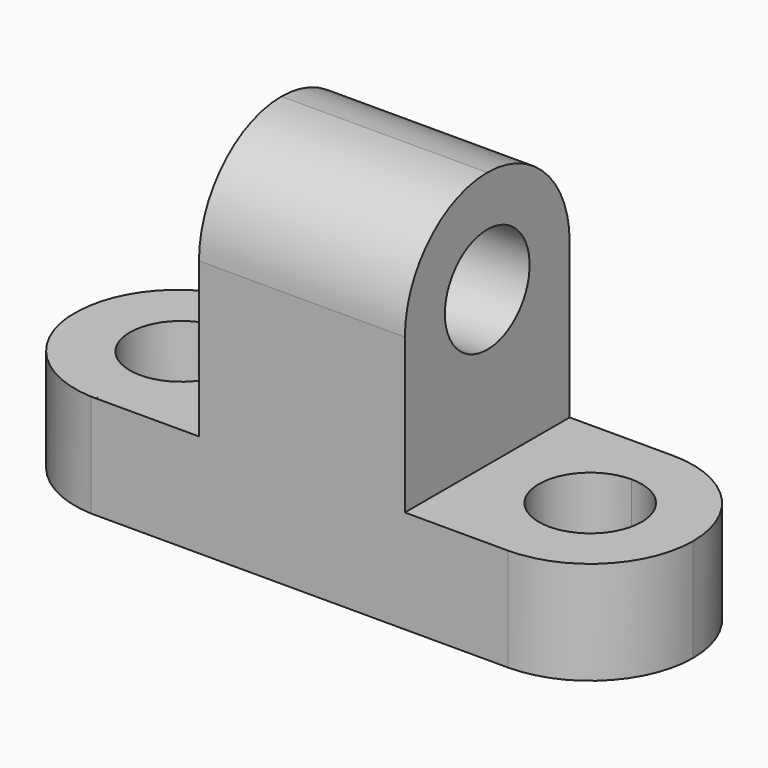
from build123d import *

# Parameters (mm, degrees)
F1_DEPTH = 25.4
F3_DEPTH = 50.801
F5_DEPTH = 12.701
F7_DEPTH = 12.701
F9_DEPTH = 12.701


with BuildPart() as f1:
    # F0 (on Front) → F1 (new body)
    with BuildSketch(Plane.XZ):
        Polygon((-38.1542058029, 12.7), (-38.1542058029, 0), (38.0457941971, 0), (38.0457941971, 12.7), (12.6457941971, 12.7), (12.6457941971, 44.45), (-12.7542058029, 44.45), (-12.7542058029, 12.7), align=None)
    extrude(amount=F1_DEPTH)

    # F2 (on face) → F3 (cut, through all)
    with BuildSketch(Plane.YZ.offset(12.6457941971)):
        with BuildLine():
            Line((-19.2294398129, 31.75), (-6.1705601871, 31.75))
            ThreePointArc((-6.1705601871, 31.75), (-12.7, 38.2794398129), (-19.2294398129, 31.75))
        make_face()
        with BuildLine():
            ThreePointArc((-19.2294398129, 31.75), (-12.7, 25.2205601871), (-6.1705601871, 31.75))
            Line((-6.1705601871, 31.75), (-19.2294398129, 31.75))
        make_face()
        with BuildLine():
            ThreePointArc((-25.4, 31.75), (-21.6802561211, 40.7302561211), (-12.7, 44.45))
            Line((-12.7, 44.45), (-25.4, 44.45))
            Line((-25.4, 44.45), (-25.4, 31.75))
        make_face()
        with BuildLine():
            ThreePointArc((-12.7, 44.45), (-3.7197438789, 40.7302561211), (0, 31.75))
            Line((0, 31.75), (0, 44.45))
            Line((0, 44.45), (-12.7, 44.45))
        make_face()
    extrude(amount=-F3_DEPTH, mode=Mode.SUBTRACT)

    # F4 (on face) → F5 (cut, through all)
    with BuildSketch(Plane.XY.offset(12.7)):
        with BuildLine():
            Line((-25.1679819405, -25.2168271691), (-25.9211060628, -25.2168271691))
            ThreePointArc((-25.9211060628, -25.2168271691), (-25.5445440017, -25.2224491047), (-25.1679819405, -25.2168271691))
        make_face()
        with BuildLine():
            ThreePointArc((25.3457941971, -6.3600277162), (19.0058219133, -12.7), (25.3457941971, -19.0399722838))
            Line((25.3457941971, -19.0399722838), (25.3457941971, -6.3600277162))
        make_face()
        with BuildLine():
            Line((25.3457941971, -6.3600277162), (25.3457941971, -19.0399722838))
            ThreePointArc((25.3457941971, -19.0399722838), (29.8288315915, -17.1830373944), (31.6857664808, -12.7))
            ThreePointArc((31.6857664808, -12.7), (29.8288315915, -8.2169626056), (25.3457941971, -6.3600277162))
        make_face()
        with BuildLine():
            Line((-25.1679819405, -18.9560678934), (-25.1679819405, -6.2607592757))
            ThreePointArc((-25.1679819405, -6.2607592757), (-31.5156362493, -12.6084135845), (-25.1679819405, -18.9560678934))
        make_face()
        with BuildLine():
            ThreePointArc((-18.8203276317, -12.6084135845), (-20.6795125341, -8.1199441781), (-25.1679819405, -6.2607592757))
            Line((-25.1679819405, -6.2607592757), (-25.1679819405, -18.9560678934))
            ThreePointArc((-25.1679819405, -18.9560678934), (-20.6795125341, -17.0968829909), (-18.8203276317, -12.6084135845))
        make_face()
        with BuildLine():
            ThreePointArc((25.3457941971, 0), (34.3260503181, -3.7197438789), (38.0457941971, -12.7))
            Line((38.0457941971, -12.7), (38.0457941971, 0))
            Line((38.0457941971, 0), (25.3457941971, 0))
        make_face()
        with BuildLine():
            ThreePointArc((38.0457941971, -12.7), (34.3260503181, -21.6802561211), (25.3457941971, -25.4))
            Line((25.3457941971, -25.4), (38.0457941971, -25.4))
            Line((38.0457941971, -25.4), (38.0457941971, -12.7))
        make_face()
    extrude(amount=-F5_DEPTH, mode=Mode.SUBTRACT)

    # F6 (on face) → F7 (cut, through all)
    with BuildSketch(Plane.XY.offset(12.7)):
        with BuildLine():
            ThreePointArc((-38.1542058029, -12.2175221546), (-34.4600291378, -3.683299298), (-25.9211060628, 0))
            Line((-25.9211060628, 0), (-38.1542058029, 0))
            Line((-38.1542058029, 0), (-38.1542058029, -12.2175221546))
        make_face()
    extrude(amount=-F7_DEPTH, mode=Mode.SUBTRACT)

    # F8 (on face) → F9 (cut, through all)
    with BuildSketch(Plane.XY.offset(12.7)):
        with BuildLine():
            Line((-38.1542058029, -25.4), (-26.090927422, -25.4))
            ThreePointArc((-26.090927422, -25.4), (-34.2975944615, -21.8697418221), (-38.1542058029, -13.8112893863))
            Line((-38.1542058029, -13.8112893863), (-38.1542058029, -25.4))
        make_face()
    extrude(amount=-F9_DEPTH, mode=Mode.SUBTRACT)


solid = f1.part
